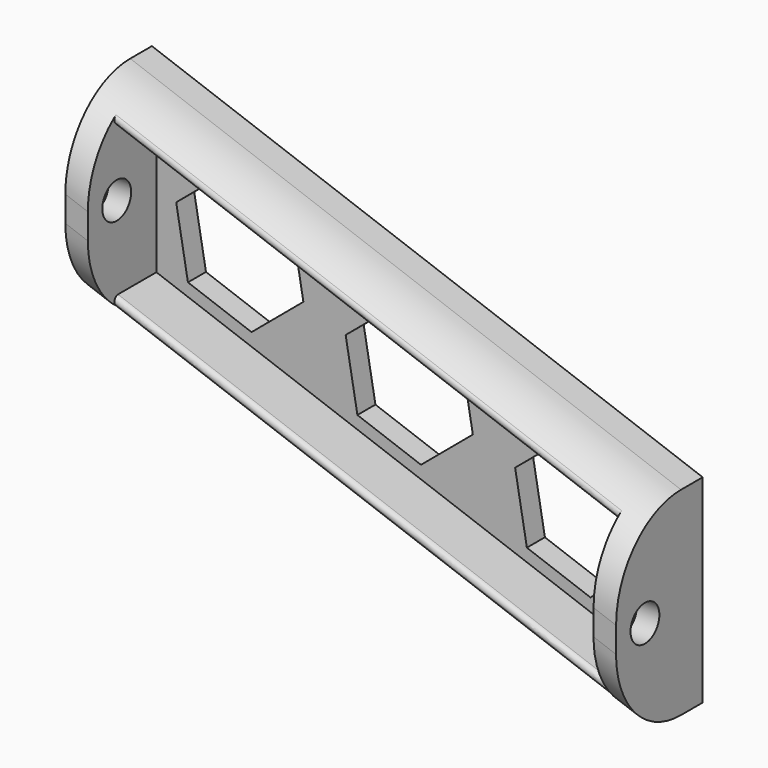
from build123d import *

# Parameters (mm, degrees)
F1_DEPTH    = 12
F2_T        = -2.5
F4_D        = 4
F4_DEPTH    = 6
F4_TIP      = 1.2017212381
F6_D        = 4
F6_DEPTH    = 6
F6_TIP      = 1.2017212381
F7_T1_DEPTH = 110
F7_T3_DEPTH = 110
F9_DEPTH    = 25
F10_R       = 0.5


# Not quite as in the source:
# - a fillet or chamfer that OpenCascade refuses, or shapes differently, is made with other operations: its cross-section is extruded or revolved along the edge and cut away or added


with BuildPart() as f1:
    # F0 (on Front) → F1 (new body)
    with BuildSketch(Plane.XZ):
        Polygon((39.4877206884, 0), (-21.5922996627, 22.2313093162), (-21.5922996627, 0.2313093162), (39.4877206884, -22), align=None)
    extrude(amount=F1_DEPTH)

    # F2
    f2_openings = [f1.faces().sort_by_distance(p)[0] for p in [
        (8.947711, -12, 0.115655),
    ]]
    offset(amount=F2_T, openings=f2_openings)

    # F4
    with Locations(Plane(origin=(-21.5922996627, 0, 0), x_dir=(0, -1, 0), z_dir=(-1, 0, 0))):
        with Locations((8, 11.2313093162)):
            Hole(F4_D / 2, depth=F4_DEPTH)
            with Locations((0, 0, -(F4_DEPTH + F4_TIP / 2))):  # 118° drill point
                Cone(0, F4_D / 2, F4_TIP, mode=Mode.SUBTRACT)

    # F6
    with Locations(Plane.YZ.offset(39.4877206884)):
        with Locations((-8, -11)):
            Hole(F6_D / 2, depth=F6_DEPTH)
            with Locations((0, 0, -(F6_DEPTH + F6_TIP / 2))):  # 118° drill point
                Cone(0, F6_D / 2, F6_TIP, mode=Mode.SUBTRACT)

    # F7: fillet of radius 9 on 2 edges, made by hand

    # F7_s2 → F7_t1 (cut)
    with BuildSketch(Plane(origin=(56.0116188142, 0, -20.3865620214), x_dir=(0, 1, 0), z_dir=(-0.9396926208, 0, 0.3420201433))):
        with BuildLine():
            ThreePointArc((-3, -13.5055958894), (-9.3639610307, -10.8695569201), (-12, -4.5055958894))
            Line((-12, -4.5055958894), (-12, -13.5055958894))
            Line((-12, -13.5055958894), (-3, -13.5055958894))
        make_face()
    extrude(amount=F7_T1_DEPTH, mode=Mode.SUBTRACT)

    # F7_s4 → F7_t3 (cut)
    with BuildSketch(Plane(origin=(-40.2839057657, 0, 14.6621426187), x_dir=(0, 1, 0), z_dir=(0.9396926208, 0, -0.3420201433))):
        with BuildLine():
            ThreePointArc((-12, 1.8323582321), (-9.3639610307, -4.5316027985), (-3, -7.1676417679))
            Line((-3, -7.1676417679), (-12, -7.1676417679))
            Line((-12, -7.1676417679), (-12, 1.8323582321))
        make_face()
    extrude(amount=F7_T3_DEPTH, mode=Mode.SUBTRACT)

    # F8 (on face) → F9 (cut)
    with BuildSketch(Plane.XZ.offset(2.5)):
        Polygon((-8.5428162153, -0.4354697523), (-2.7932286645, 4.389007041), (-4.0965543521, 11.7805343179), (-11.1494675905, 14.3475848015), (-16.8990551413, 9.5231080082), (-15.5957294537, 2.1315807313), align=None)
        Polygon((10.2510362004, -7.2758726188), (16.0006237512, -2.4513958255), (14.6972980636, 4.9401314514), (7.6443848253, 7.507181935), (1.8947972745, 2.6827051417), (3.198122962, -4.7088221352), align=None)
        Polygon((29.0448886161, -14.1162754854), (34.7944761669, -9.2917986921), (33.4911504793, -1.9002714151), (26.438237241, 0.6667790685), (20.6886496902, -4.1576977248), (21.9919753777, -11.5492250017), align=None)
    extrude(amount=-F9_DEPTH, mode=Mode.SUBTRACT)

    # F10
    f10_edges = [f1.edges().sort_by_distance(p)[0] for p in [
        (8.947711, -9.22495, -8.223901),
        (8.947711, -9.22495, 8.45521),
    ]]
    fillet(f10_edges, radius=F10_R)


solid = f1.part
